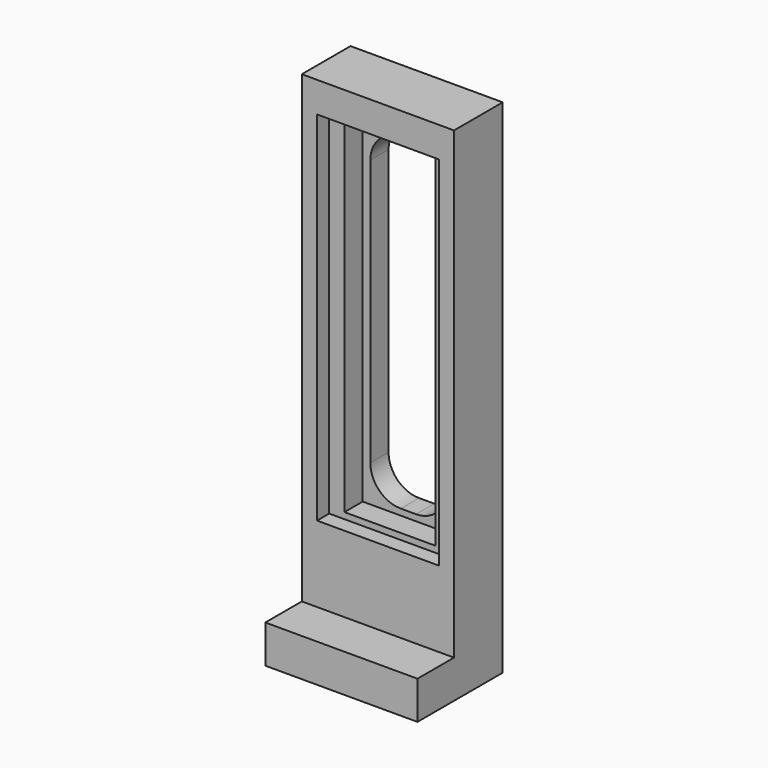
from build123d import *

# Parameters (mm, degrees)
F0_W     = 254
F0_H     = 774.7
F0_W_2   = 203.2
F0_H_2   = 596.9
F0_W_3   = 152.4
F0_H_3   = 571.5
F0_W_4   = 127
F0_H_4   = 546.1
F0_H_5   = 63.5
F1_DEPTH = 101.6
F2_DEPTH = 25.4
F3_DEPTH = 63.5
F4_R     = 50.8
F5_DEPTH = 76.2


# Not quite as in the source:
# - a feature names something its author has since deleted; it is built from what else it names


with BuildPart() as f1:
    # F0 (on Front) → F1 (new body)
    with BuildSketch(Plane.XZ):
        with Locations((0, 260.35)):
            Rectangle(F0_W, F0_H)
        with Locations((0, 298.45)):
            Rectangle(F0_W_2, F0_H_2, mode=Mode.SUBTRACT)
        with Locations((0, 298.45)):
            Rectangle(F0_W_2, F0_H_2)
        with Locations((0, 296.15)):
            Rectangle(F0_W_3, F0_H_3, mode=Mode.SUBTRACT)
        with Locations((0, 296.15)):
            Rectangle(F0_W_3, F0_H_3)
        with Locations((0, 293.85)):
            Rectangle(F0_W_4, F0_H_4, mode=Mode.SUBTRACT)
        with Locations((0, -158.75)):
            Rectangle(F0_W, F0_H_5)
    extrude(amount=-F1_DEPTH)

    # F0 (on Front) → F2 (cut)
    with BuildSketch(Plane.XZ):
        with Locations((0, 298.45)):
            Rectangle(F0_W_2, F0_H_2)
        with Locations((0, 296.15)):
            Rectangle(F0_W_3, F0_H_3, mode=Mode.SUBTRACT)
    extrude(amount=-F2_DEPTH, mode=Mode.SUBTRACT)

    # F0 (on Front) → F3 (cut)
    with BuildSketch(Plane.XZ):
        with Locations((0, 296.15)):
            Rectangle(F0_W_3, F0_H_3)
        with Locations((0, 293.85)):
            Rectangle(F0_W_4, F0_H_4, mode=Mode.SUBTRACT)
    extrude(amount=-F3_DEPTH, mode=Mode.SUBTRACT)

    # F4
    f4_edges = [f1.edges().sort_by_distance(p)[0] for p in [
        (63.5, 82.55, 566.9),
        (-63.5, 82.55, 566.9),
        (-63.5, 82.55, 20.8),
        (63.5, 82.55, 20.8),
    ]]
    fillet(f4_edges, radius=F4_R)

    # F0 (on Front) → F5 (join)
    with BuildSketch(Plane.XZ):
        with Locations((0, -158.75)):
            Rectangle(F0_W, F0_H_5)
    extrude(amount=F5_DEPTH)


solid = f1.part
